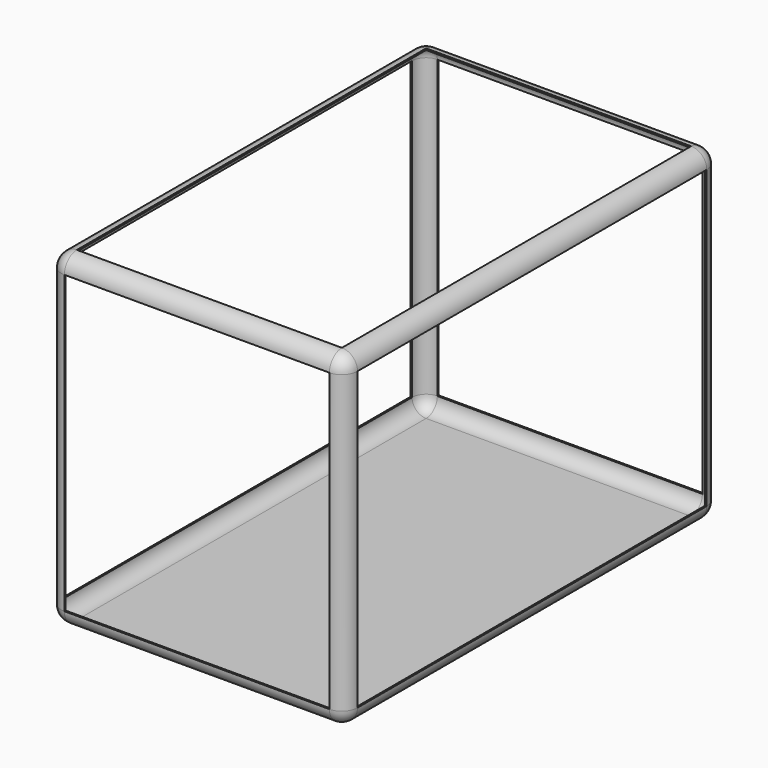
from build123d import *

# Parameters (mm, degrees)
F0_W     = 482.6
F0_H     = 533.4
F1_DEPTH = 762
F2_R     = 25.4
F3_T     = -2.54


# Not quite as in the source:
# - a shell that OpenCascade refuses in one call is made with other operations: the cavity is built on its own and cut out


with BuildPart() as f1:
    # F0 (on Front) → F1 (new body)
    with BuildSketch(Plane.XZ):
        with Locations((241.3, 266.7)):
            Rectangle(F0_W, F0_H)
    extrude(amount=F1_DEPTH)

    # F2
    f2_edges = [f1.edges().sort_by_distance(p)[0] for p in [
        (482.6, -381, 533.4),
        (482.6, -762, 266.7),
        (0, -381, 533.4),
        (241.3, 0, 533.4),
        (241.3, -762, 533.4),
        (241.3, -762, 0),
        (482.6, -381, 0),
        (482.6, 0, 266.7),
        (0, 0, 266.7),
        (241.3, 0, 0),
        (0, -381, 0),
        (0, -762, 266.7),
    ]]
    fillet(f2_edges, radius=F2_R)

    # F3: a shell. OpenCascade refuses it in one call, so the cavity is built on its own and cut out:
    # the body offset inwards by the wall thickness, plus a prism from it out through each open face.
    f3_core = offset(f1.part, amount=F3_T, mode=Mode.PRIVATE)
    f3_exits = [f3_core.faces().sort_by_distance(p)[0] for p in [
        (241.3, -2.54, 266.7),
        (241.3, -759.46, 266.7),
        (480.06, -381, 266.7),
        (241.3, -381, 530.86),
        (2.54, -381, 266.7),
    ]]
    add(f3_core, mode=Mode.SUBTRACT)
    extrude(f3_exits, amount=-F3_T, mode=Mode.SUBTRACT)


solid = f1.part
